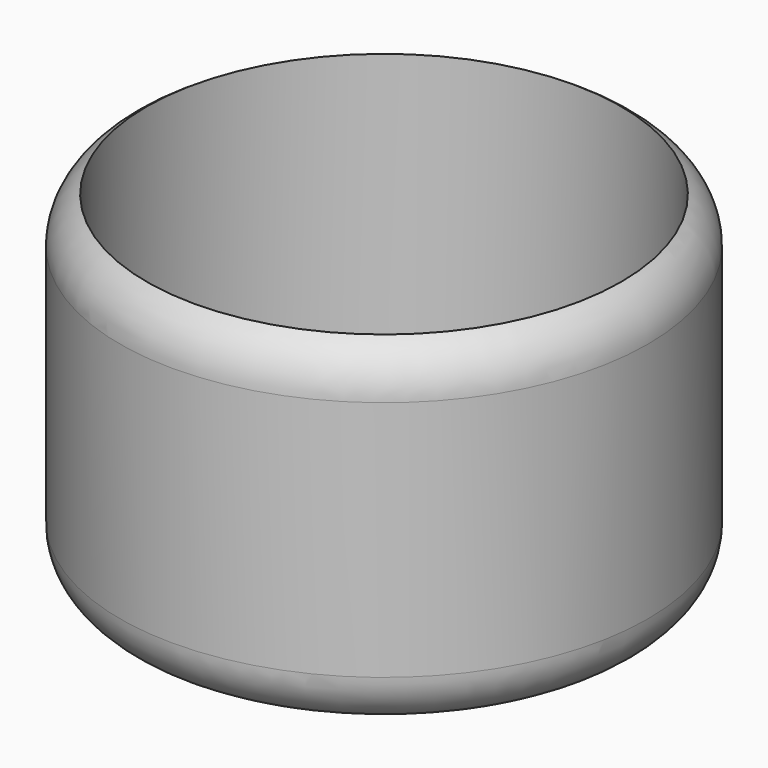
from build123d import *

# Parameters (mm, degrees)
F0_R     = 25.1418135505
F1_DEPTH = 32.512
F2_T     = -2.54


# Not quite as in the source:
# - a fillet or chamfer that OpenCascade refuses, or shapes differently, is made with other operations: its cross-section is extruded or revolved along the edge and cut away or added


with BuildPart() as f1:
    # F0 (on Top) → F1 (new body)
    with BuildSketch(Plane.XY):
        Circle(F0_R)
    extrude(amount=F1_DEPTH)

    # F2
    f2_openings = [f1.faces().sort_by_distance(p)[0] for p in [
        (0, 0, 32.512),
    ]]
    offset(amount=F2_T, openings=f2_openings)

    # F3: fillet of radius 5.08 on 3 edges, made by hand

    # F3_s1 → F3_t2 (revolve, cut)
    with BuildSketch(Plane.XZ):
        with BuildLine():
            ThreePointArc((25.1418135505, 28.1125909488), (24.4612226018, 30.6525909488), (22.6018135505, 32.512))
            Line((22.6018135505, 32.512), (22.6526135505, 32.599988181))
            ThreePointArc((22.6526135505, 32.599988181), (23.8718135505, 32.6136), (25.1418135505, 32.6136))
            Line((25.1418135505, 32.6136), (25.2434135505, 32.512))
            Line((25.2434135505, 32.512), (25.2434135505, 28.1125909488))
            Line((25.2434135505, 28.1125909488), (25.1418135505, 28.1125909488))
        make_face()
    revolve(axis=Axis((0, 0, 32.512), (0, 0, 1)), mode=Mode.SUBTRACT)

    # F3_s3 → F3_t4 (revolve, cut)
    with BuildSketch(Plane.XZ):
        with BuildLine():
            ThreePointArc((25.1418135505, 5.08), (23.653915999, 1.4878975516), (20.0618135505, 0))
            Line((20.0618135505, 0), (20.0618135505, -0.1016))
            Line((20.0618135505, -0.1016), (25.2434135505, -0.1016))
            Line((25.2434135505, -0.1016), (25.2434135505, 5.08))
            Line((25.2434135505, 5.08), (25.1418135505, 5.08))
        make_face()
    revolve(axis=Axis((0, 0, 0), (0, 0, 1)), mode=Mode.SUBTRACT)


solid = f1.part
